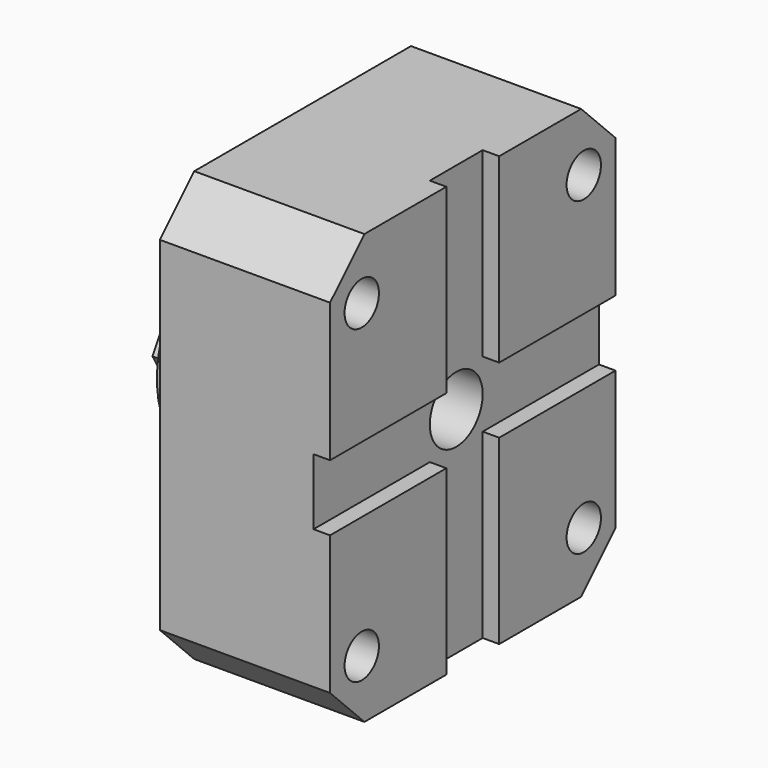
from build123d import *

# Parameters (mm, degrees)
F0_W      = 108
F0_H      = 130
F1_DEPTH  = 51.5
F2_R      = 6.5
F3_DEPTH  = 51.501
F4_R      = 10
F5_DEPTH  = 20
F7_R      = 32
F8_DEPTH  = 18.5
F10_DEPTH = 8
F11_R     = 10
F12_DEPTH = 78.001
F13_SIZE  = 13
F14_W     = 20
F14_H     = 55
F14_H_2   = 20
F14_W_2   = 44
F15_DEPTH = 5


with BuildPart() as f1:
    # F0 (on Right) → F1 (new body)
    with BuildSketch(Plane.YZ):
        Rectangle(F0_W, F0_H)
    extrude(amount=-F1_DEPTH)

    # F2 (on face) → F3 (cut, through all)
    with BuildSketch(Plane(origin=(-51.5, 0, 0), x_dir=(0, -1, 0), z_dir=(-1, 0, 0))):
        with Locations((42, 47)):
            Circle(F2_R)
        with Locations((-42, 47)):
            Circle(F2_R)
        with Locations((-42, -47)):
            Circle(F2_R)
        with Locations((42, -47)):
            Circle(F2_R)
    extrude(amount=-F3_DEPTH, mode=Mode.SUBTRACT)

    # F4 (on face) → F5 (cut)
    with BuildSketch(Plane(origin=(-51.5, 0, 0), x_dir=(0, -1, 0), z_dir=(-1, 0, 0))):
        with Locations((-42, 47)):
            Circle(F4_R)
        with Locations((-42, -47)):
            Circle(F4_R)
        with Locations((42, 47)):
            Circle(F4_R)
        with Locations((42, -47)):
            Circle(F4_R)
    extrude(amount=-F5_DEPTH, mode=Mode.SUBTRACT)

    # F7 (on offset) → F8 (join, through all)
    with BuildSketch(Plane.YZ.offset(-70)):
        Circle(F7_R)
    extrude(amount=F8_DEPTH)

    # F9 (on face) → F10 (join)
    with BuildSketch(Plane(origin=(-70, 0, 0), x_dir=(0, -1, 0), z_dir=(-1, 0, 0))):
        Polygon((23.6713610368, 0), (11.8356805184, 20.5), (-11.8356805184, 20.5), (-23.6713610368, 0), (-11.8356805184, -20.5), (11.8356805184, -20.5), align=None)
    extrude(amount=F10_DEPTH)

    # F11 (on face) → F12 (cut, through all)
    with BuildSketch(Plane(origin=(-78, 0, 0), x_dir=(0, -1, 0), z_dir=(-1, 0, 0))):
        Circle(F11_R)
    extrude(amount=-F12_DEPTH, mode=Mode.SUBTRACT)

    # F13
    f13_edges = [f1.edges().sort_by_distance(p)[0] for p in [
        (-25.75, -54, 65),
        (-25.75, 54, 65),
        (-25.75, -54, -65),
        (-25.75, 54, -65),
    ]]
    chamfer(f13_edges, length=F13_SIZE)

    # F14 (on face) → F15 (cut)
    with BuildSketch(Plane.YZ):
        with Locations((0, 37.5)):
            Rectangle(F14_W, F14_H)
        Rectangle(F14_W, F14_H_2)
        with Locations((-32, 0)):
            Rectangle(F14_W_2, F14_H_2)
        with Locations((32, 0)):
            Rectangle(F14_W_2, F14_H_2)
        with Locations((0, -37.5)):
            Rectangle(F14_W, F14_H)
    extrude(amount=-F15_DEPTH, mode=Mode.SUBTRACT)


solid = f1.part
